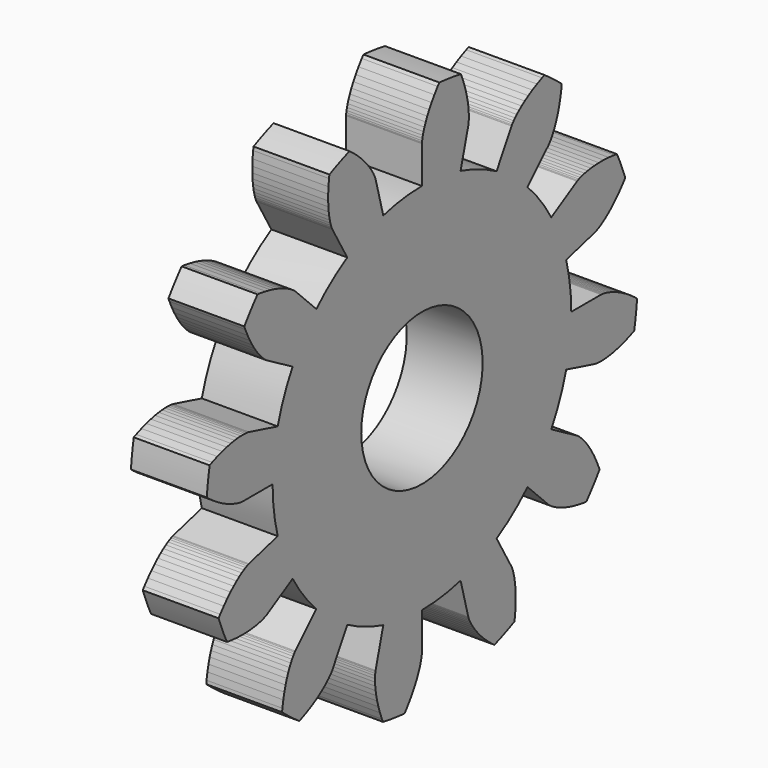
from build123d import *

# Parameters (mm, degrees)
F2_DEPTH = 5
F3_R     = 5
F4_DEPTH = 5.001


# Not quite as in the source:
# - a feature names something its author has since deleted; it is built from what else it names


with BuildPart() as f2:
    # F1 (on Right) → F2 (new body)
    with BuildSketch(Plane.YZ):
        with BuildLine():
            ThreePointArc((11.8820660929, -3.183790014), (12.1959813576, -1.6056314063), (12.30122, 0))
            ThreePointArc((12.30122, 0), (12.1959813576, 1.6056314063), (11.8820660929, 3.183790014))
            ThreePointArc((11.8820660929, 3.183790014), (11.3648453829, 4.7074730919), (10.6531690175, 6.15061))
            ThreePointArc((10.6531690175, 6.15061), (9.7592139767, 7.4885082658), (8.6982760789, 8.6982760789))
            ThreePointArc((8.6982760789, 8.6982760789), (7.4885082658, 9.7592139767), (6.15061, 10.6531690175))
            ThreePointArc((6.15061, 10.6531690175), (4.7074730919, 11.3648453829), (3.183790014, 11.8820660929))
            ThreePointArc((3.183790014, 11.8820660929), (1.6056314063, 12.1959813576), (0, 12.30122))
            ThreePointArc((0, 12.30122), (-1.6056314063, 12.1959813576), (-3.183790014, 11.8820660929))
            ThreePointArc((-3.183790014, 11.8820660929), (-4.7074730919, 11.3648453829), (-6.15061, 10.6531690175))
            ThreePointArc((-6.15061, 10.6531690175), (-7.4885082658, 9.7592139767), (-8.6982760789, 8.6982760789))
            ThreePointArc((-8.6982760789, 8.6982760789), (-9.7592139767, 7.4885082658), (-10.6531690175, 6.15061))
            ThreePointArc((-10.6531690175, 6.15061), (-11.3648453829, 4.7074730919), (-11.8820660929, 3.183790014))
            ThreePointArc((-11.8820660929, 3.183790014), (-12.1959813576, 1.6056314063), (-12.30122, 0))
            ThreePointArc((-12.30122, 0), (-12.1959813576, -1.6056314063), (-11.8820660929, -3.183790014))
            ThreePointArc((-11.8820660929, -3.183790014), (-11.3648453829, -4.7074730919), (-10.6531690175, -6.15061))
            ThreePointArc((-10.6531690175, -6.15061), (-9.7592139767, -7.4885082658), (-8.6982760789, -8.6982760789))
            ThreePointArc((-8.6982760789, -8.6982760789), (-7.4885082658, -9.7592139767), (-6.15061, -10.6531690175))
            ThreePointArc((-6.15061, -10.6531690175), (-4.7074730919, -11.3648453829), (-3.183790014, -11.8820660929))
            ThreePointArc((-3.183790014, -11.8820660929), (-1.6056314063, -12.1959813576), (0, -12.30122))
            ThreePointArc((0, -12.30122), (1.6056314063, -12.1959813576), (3.183790014, -11.8820660929))
            ThreePointArc((3.183790014, -11.8820660929), (4.7074730919, -11.3648453829), (6.15061, -10.6531690175))
            ThreePointArc((6.15061, -10.6531690175), (7.4885082658, -9.7592139767), (8.6982760789, -8.6982760789))
            ThreePointArc((8.6982760789, -8.6982760789), (9.7592139767, -7.4885082658), (10.6531690175, -6.15061))
            ThreePointArc((10.6531690175, -6.15061), (11.3648453829, -4.7074730919), (11.8820660929, -3.183790014))
        make_face()
        with BuildLine():
            Line((-12.777832476, -7.3772850197), (-10.6531690175, -6.15061))
            ThreePointArc((-10.6531690175, -6.15061), (-11.3648453829, -4.7074730919), (-11.8820660929, -3.183790014))
            Line((-11.8820660929, -3.183790014), (-14.2518202568, -3.8187637285))
            Line((-14.2518202568, -3.8187637285), (-14.2694648269, -3.824127867))
            Line((-14.2694648269, -3.824127867), (-14.3216296662, -3.8425556758))
            Line((-14.3216296662, -3.8425556758), (-14.4069660463, -3.8774806861))
            Line((-14.4069660463, -3.8774806861), (-14.5238699427, -3.9322299545))
            Line((-14.5238699427, -3.9322299545), (-14.6704895203, -4.0100072128))
            Line((-14.6704895203, -4.0100072128), (-14.84473366, -4.1138765105))
            Line((-14.84473366, -4.1138765105), (-15.0442814965, -4.2467464121))
            Line((-15.0442814965, -4.2467464121), (-15.2665929313, -4.4113548082))
            Line((-15.2665929313, -4.4113548082), (-15.5089200841, -4.6102543989))
            Line((-15.5089200841, -4.6102543989), (-15.7683196404, -4.8457989047))
            Line((-15.7683196404, -4.8457989047), (-16.0416660512, -5.1201300574))
            Line((-16.0416660512, -5.1201300574), (-16.3256655366, -5.4351654226))
            Line((-16.3256655366, -5.4351654226), (-16.616870844, -5.7925870994))
            Line((-16.616870844, -5.7925870994), (-16.7475876092, -5.9704865189))
            ThreePointArc((-16.7475876092, -5.9704865189), (-16.4265780881, -6.8041114275), (-16.0641042715, -7.6205612624))
            Line((-16.0641042715, -7.6205612624), (-15.8458796744, -7.6539244373))
            Line((-15.8458796744, -7.6539244373), (-15.3872311355, -7.7007464811))
            Line((-15.3872311355, -7.7007464811), (-14.9636495305, -7.7226921621))
            Line((-14.9636495305, -7.7226921621), (-14.5763830115, -7.7233884799))
            Line((-14.5763830115, -7.7233884799), (-14.2264047088, -7.7065204119))
            Line((-14.2264047088, -7.7065204119), (-13.9144102864, -7.6758124883))
            Line((-13.9144102864, -7.6758124883), (-13.6408166502, -7.6350102783))
            Line((-13.6408166502, -7.6350102783), (-13.4057618135, -7.5878618584))
            Line((-13.4057618135, -7.5878618584), (-13.2091059159, -7.5380993303))
            Line((-13.2091059159, -7.5380993303), (-13.0504333916, -7.4894204595))
            Line((-13.0504333916, -7.4894204595), (-12.9290562747, -7.4454705006))
            Line((-12.9290562747, -7.4454705006), (-12.84401863, -7.4098242792))
            Line((-12.84401863, -7.4098242792), (-12.7941020899, -7.3859685961))
            Line((-12.7941020899, -7.3859685961), (-12.777832476, -7.3772850197))
        make_face()
        with BuildLine():
            Line((-7.3772850197, -12.777832476), (-6.15061, -10.6531690175))
            ThreePointArc((-6.15061, -10.6531690175), (-7.4885082658, -9.7592139767), (-8.6982760789, -8.6982760789))
            Line((-8.6982760789, -8.6982760789), (-10.4330565283, -10.4330565283))
            Line((-10.4330565283, -10.4330565283), (-10.445655105, -10.4465242936))
            Line((-10.445655105, -10.4465242936), (-10.4816172766, -10.4885656638))
            Line((-10.4816172766, -10.4885656638), (-10.5380582445, -10.5614798))
            Line((-10.5380582445, -10.5614798), (-10.6119253544, -10.6673460055))
            Line((-10.6119253544, -10.6673460055), (-10.7000130041, -10.8080128758))
            Line((-10.7000130041, -10.8080128758), (-10.7989782067, -10.9850883961))
            Line((-10.7989782067, -10.9850883961), (-10.9053567516, -11.1999310245))
            Line((-10.9053567516, -11.1999310245), (-11.0155799037, -11.4536417946))
            Line((-11.0155799037, -11.4536417946), (-11.1259915786, -11.7470574694))
            Line((-11.1259915786, -11.7470574694), (-11.2328659313, -12.0807447733))
            Line((-11.2328659313, -12.0807447733), (-11.3324252906, -12.454995726))
            Line((-11.3324252906, -12.454995726), (-11.4208583771, -12.869824098))
            Line((-11.4208583771, -12.869824098), (-11.4943387326, -13.3249630037))
            Line((-11.4943387326, -13.3249630037), (-11.5185930622, -13.5443868029))
            ThreePointArc((-11.5185930622, -13.5443868029), (-10.8237782078, -14.1058223904), (-10.1016417569, -14.6316517801))
            Line((-10.1016417569, -14.6316517801), (-9.8959721247, -14.5514328385))
            Line((-9.8959721247, -14.5514328385), (-9.4753598166, -14.3626576485))
            Line((-9.4753598166, -14.3626576485), (-9.0975545457, -14.1698723633))
            Line((-9.0975545457, -14.1698723633), (-8.7618237433, -13.9768421326))
            Line((-8.7618237433, -13.9768421326), (-8.4671676764, -13.7872448059))
            Line((-8.4671676764, -13.7872448059), (-8.2123265426, -13.6046537527))
            Line((-8.2123265426, -13.6046537527), (-7.9957886083, -13.4325211843))
            Line((-7.9957886083, -13.4325211843), (-7.8157993584, -13.2741620365))
            Line((-7.8157993584, -13.2741620365), (-7.6703716193, -13.1327384743))
            Line((-7.6703716193, -13.1327384743), (-7.5572966178, -13.0112450734))
            Line((-7.5572966178, -13.0112450734), (-7.4741559306, -12.912494734))
            Line((-7.4741559306, -12.912494734), (-7.4183342807, -12.8391053784))
            Line((-7.4183342807, -12.8391053784), (-7.3870331304, -12.7934874807))
            Line((-7.3870331304, -12.7934874807), (-7.3772850197, -12.777832476))
        make_face()
        with BuildLine():
            Line((0, -14.7545700394), (0, -12.30122))
            ThreePointArc((0, -12.30122), (-1.6056314063, -12.1959813576), (-3.183790014, -11.8820660929))
            Line((-3.183790014, -11.8820660929), (-3.8187637285, -14.2518202568))
            Line((-3.8187637285, -14.2518202568), (-3.8229405333, -14.269782972))
            Line((-3.8229405333, -14.269782972), (-3.8330640024, -14.3241729524))
            Line((-3.8330640024, -14.3241729524), (-3.8454862463, -14.4155389306))
            Line((-3.8454862463, -14.4155389306), (-3.8565239372, -14.5441553089))
            Line((-3.8565239372, -14.5441553089), (-3.8624766445, -14.7100202169))
            Line((-3.8624766445, -14.7100202169), (-3.8596452639, -14.9128547172))
            Line((-3.8596452639, -14.9128547172), (-3.844350472, -15.1521031637))
            Line((-3.844350472, -15.1521031637), (-3.8129511367, -15.4269347118))
            Line((-3.8129511367, -15.4269347118), (-3.7618626147, -15.7362459776))
            Line((-3.7618626147, -15.7362459776), (-3.6875748671, -16.078664836))
            Line((-3.6875748671, -16.078664836), (-3.5866703252, -16.4525553481))
            Line((-3.5866703252, -16.4525553481), (-3.4558414386, -16.8560237997))
            Line((-3.4558414386, -16.8560237997), (-3.2919078403, -17.286925832))
            Line((-3.2919078403, -17.286925832), (-3.2032008062, -17.4890795811))
            ThreePointArc((-3.2032008062, -17.4890795811), (-2.3207556977, -17.6278896352), (-1.4324524914, -17.7222030194))
            Line((-1.4324524914, -17.7222030194), (-1.2944468359, -17.549896562))
            Line((-1.2944468359, -17.549896562), (-1.024573487, -17.1761062978))
            Line((-1.024573487, -17.1761062978), (-0.7937771672, -16.8202467078))
            Line((-0.7937771672, -16.8202467078), (-0.5995408789, -16.4852122232))
            Line((-0.5995408789, -16.4852122232), (-0.439159903, -16.1736880883))
            Line((-0.439159903, -16.1736880883), (-0.3097565337, -15.8881390309))
            Line((-0.3097565337, -15.8881390309), (-0.208295466, -15.6307988866))
            Line((-0.208295466, -15.6307988866), (-0.131599777, -15.4036612167))
            Line((-0.131599777, -15.4036612167), (-0.0763674416, -15.2084709496))
            Line((-0.0763674416, -15.2084709496), (-0.0391883182, -15.0467170773))
            Line((-0.0391883182, -15.0467170773), (-0.0165615407, -14.9196264312))
            Line((-0.0165615407, -14.9196264312), (-0.0049132517, -14.8281585599))
            Line((-0.0049132517, -14.8281585599), (-0.0006146092, -14.7730017265))
            Line((-0.0006146092, -14.7730017265), (0, -14.7545700394))
        make_face()
        with BuildLine():
            Line((7.3772850197, -12.777832476), (6.15061, -10.6531690175))
            ThreePointArc((6.15061, -10.6531690175), (4.7074730919, -11.3648453829), (3.183790014, -11.8820660929))
            Line((3.183790014, -11.8820660929), (3.8187637285, -14.2518202568))
            Line((3.8187637285, -14.2518202568), (3.824127867, -14.2694648269))
            Line((3.824127867, -14.2694648269), (3.8425556758, -14.3216296662))
            Line((3.8425556758, -14.3216296662), (3.8774806861, -14.4069660463))
            Line((3.8774806861, -14.4069660463), (3.9322299545, -14.5238699427))
            Line((3.9322299545, -14.5238699427), (4.0100072128, -14.6704895203))
            Line((4.0100072128, -14.6704895203), (4.1138765105, -14.84473366))
            Line((4.1138765105, -14.84473366), (4.2467464121, -15.0442814965))
            Line((4.2467464121, -15.0442814965), (4.4113548082, -15.2665929313))
            Line((4.4113548082, -15.2665929313), (4.6102543989, -15.5089200841))
            Line((4.6102543989, -15.5089200841), (4.8457989047, -15.7683196404))
            Line((4.8457989047, -15.7683196404), (5.1201300574, -16.0416660512))
            Line((5.1201300574, -16.0416660512), (5.4351654226, -16.3256655366))
            Line((5.4351654226, -16.3256655366), (5.7925870994, -16.616870844))
            Line((5.7925870994, -16.616870844), (5.9704865189, -16.7475876092))
            ThreePointArc((5.9704865189, -16.7475876092), (6.8041114275, -16.4265780881), (7.6205612624, -16.0641042715))
            Line((7.6205612624, -16.0641042715), (7.6539244373, -15.8458796744))
            Line((7.6539244373, -15.8458796744), (7.7007464811, -15.3872311355))
            Line((7.7007464811, -15.3872311355), (7.7226921621, -14.9636495305))
            Line((7.7226921621, -14.9636495305), (7.7233884799, -14.5763830115))
            Line((7.7233884799, -14.5763830115), (7.7065204119, -14.2264047088))
            Line((7.7065204119, -14.2264047088), (7.6758124883, -13.9144102864))
            Line((7.6758124883, -13.9144102864), (7.6350102783, -13.6408166502))
            Line((7.6350102783, -13.6408166502), (7.5878618584, -13.4057618135))
            Line((7.5878618584, -13.4057618135), (7.5380993303, -13.2091059159))
            Line((7.5380993303, -13.2091059159), (7.4894204595, -13.0504333916))
            Line((7.4894204595, -13.0504333916), (7.4454705006, -12.9290562747))
            Line((7.4454705006, -12.9290562747), (7.4098242792, -12.84401863))
            Line((7.4098242792, -12.84401863), (7.3859685961, -12.7941020899))
            Line((7.3859685961, -12.7941020899), (7.3772850197, -12.777832476))
        make_face()
        with BuildLine():
            Line((12.777832476, -7.3772850197), (10.6531690175, -6.15061))
            ThreePointArc((10.6531690175, -6.15061), (9.7592139767, -7.4885082658), (8.6982760789, -8.6982760789))
            Line((8.6982760789, -8.6982760789), (10.4330565283, -10.4330565283))
            Line((10.4330565283, -10.4330565283), (10.4465242936, -10.445655105))
            Line((10.4465242936, -10.445655105), (10.4885656638, -10.4816172766))
            Line((10.4885656638, -10.4816172766), (10.5614798, -10.5380582445))
            Line((10.5614798, -10.5380582445), (10.6673460055, -10.6119253544))
            Line((10.6673460055, -10.6119253544), (10.8080128758, -10.7000130041))
            Line((10.8080128758, -10.7000130041), (10.9850883961, -10.7989782067))
            Line((10.9850883961, -10.7989782067), (11.1999310245, -10.9053567516))
            Line((11.1999310245, -10.9053567516), (11.4536417946, -11.0155799037))
            Line((11.4536417946, -11.0155799037), (11.7470574694, -11.1259915786))
            Line((11.7470574694, -11.1259915786), (12.0807447733, -11.2328659313))
            Line((12.0807447733, -11.2328659313), (12.454995726, -11.3324252906))
            Line((12.454995726, -11.3324252906), (12.869824098, -11.4208583771))
            Line((12.869824098, -11.4208583771), (13.3249630037, -11.4943387326))
            Line((13.3249630037, -11.4943387326), (13.5443868029, -11.5185930622))
            ThreePointArc((13.5443868029, -11.5185930622), (14.1058223904, -10.8237782078), (14.6316517801, -10.1016417569))
            Line((14.6316517801, -10.1016417569), (14.5514328385, -9.8959721247))
            Line((14.5514328385, -9.8959721247), (14.3626576485, -9.4753598166))
            Line((14.3626576485, -9.4753598166), (14.1698723633, -9.0975545457))
            Line((14.1698723633, -9.0975545457), (13.9768421326, -8.7618237433))
            Line((13.9768421326, -8.7618237433), (13.7872448059, -8.4671676764))
            Line((13.7872448059, -8.4671676764), (13.6046537527, -8.2123265426))
            Line((13.6046537527, -8.2123265426), (13.4325211843, -7.9957886083))
            Line((13.4325211843, -7.9957886083), (13.2741620365, -7.8157993584))
            Line((13.2741620365, -7.8157993584), (13.1327384743, -7.6703716193))
            Line((13.1327384743, -7.6703716193), (13.0112450734, -7.5572966178))
            Line((13.0112450734, -7.5572966178), (12.912494734, -7.4741559306))
            Line((12.912494734, -7.4741559306), (12.8391053784, -7.4183342807))
            Line((12.8391053784, -7.4183342807), (12.7934874807, -7.3870331304))
            Line((12.7934874807, -7.3870331304), (12.777832476, -7.3772850197))
        make_face()
        with BuildLine():
            Line((14.7545700394, 0), (12.30122, 0))
            ThreePointArc((12.30122, 0), (12.1959813576, -1.6056314063), (11.8820660929, -3.183790014))
            Line((11.8820660929, -3.183790014), (14.2518202568, -3.8187637285))
            Line((14.2518202568, -3.8187637285), (14.269782972, -3.8229405333))
            Line((14.269782972, -3.8229405333), (14.3241729524, -3.8330640024))
            Line((14.3241729524, -3.8330640024), (14.4155389306, -3.8454862463))
            Line((14.4155389306, -3.8454862463), (14.5441553089, -3.8565239372))
            Line((14.5441553089, -3.8565239372), (14.7100202169, -3.8624766445))
            Line((14.7100202169, -3.8624766445), (14.9128547172, -3.8596452639))
            Line((14.9128547172, -3.8596452639), (15.1521031637, -3.844350472))
            Line((15.1521031637, -3.844350472), (15.4269347118, -3.8129511367))
            Line((15.4269347118, -3.8129511367), (15.7362459776, -3.7618626147))
            Line((15.7362459776, -3.7618626147), (16.078664836, -3.6875748671))
            Line((16.078664836, -3.6875748671), (16.4525553481, -3.5866703252))
            Line((16.4525553481, -3.5866703252), (16.8560237997, -3.4558414386))
            Line((16.8560237997, -3.4558414386), (17.286925832, -3.2919078403))
            Line((17.286925832, -3.2919078403), (17.4890795811, -3.2032008062))
            ThreePointArc((17.4890795811, -3.2032008062), (17.6278896352, -2.3207556977), (17.7222030194, -1.4324524914))
            Line((17.7222030194, -1.4324524914), (17.549896562, -1.2944468359))
            Line((17.549896562, -1.2944468359), (17.1761062978, -1.024573487))
            Line((17.1761062978, -1.024573487), (16.8202467078, -0.7937771672))
            Line((16.8202467078, -0.7937771672), (16.4852122232, -0.5995408789))
            Line((16.4852122232, -0.5995408789), (16.1736880883, -0.439159903))
            Line((16.1736880883, -0.439159903), (15.8881390309, -0.3097565337))
            Line((15.8881390309, -0.3097565337), (15.6307988866, -0.208295466))
            Line((15.6307988866, -0.208295466), (15.4036612167, -0.131599777))
            Line((15.4036612167, -0.131599777), (15.2084709496, -0.0763674416))
            Line((15.2084709496, -0.0763674416), (15.0467170773, -0.0391883182))
            Line((15.0467170773, -0.0391883182), (14.9196264312, -0.0165615407))
            Line((14.9196264312, -0.0165615407), (14.8281585599, -0.0049132517))
            Line((14.8281585599, -0.0049132517), (14.7730017265, -0.0006146092))
            Line((14.7730017265, -0.0006146092), (14.7545700394, 0))
        make_face()
        with BuildLine():
            ThreePointArc((10.6531690175, 6.15061), (11.3648453829, 4.7074730919), (11.8820660929, 3.183790014))
            Line((11.8820660929, 3.183790014), (14.2518202568, 3.8187637285))
            Line((14.2518202568, 3.8187637285), (14.2694648269, 3.824127867))
            Line((14.2694648269, 3.824127867), (14.3216296662, 3.8425556758))
            Line((14.3216296662, 3.8425556758), (14.4069660463, 3.8774806861))
            Line((14.4069660463, 3.8774806861), (14.5238699427, 3.9322299545))
            Line((14.5238699427, 3.9322299545), (14.6704895203, 4.0100072128))
            Line((14.6704895203, 4.0100072128), (14.84473366, 4.1138765105))
            Line((14.84473366, 4.1138765105), (15.0442814965, 4.2467464121))
            Line((15.0442814965, 4.2467464121), (15.2665929313, 4.4113548082))
            Line((15.2665929313, 4.4113548082), (15.5089200841, 4.6102543989))
            Line((15.5089200841, 4.6102543989), (15.7683196404, 4.8457989047))
            Line((15.7683196404, 4.8457989047), (16.0416660512, 5.1201300574))
            Line((16.0416660512, 5.1201300574), (16.3256655366, 5.4351654226))
            Line((16.3256655366, 5.4351654226), (16.616870844, 5.7925870994))
            Line((16.616870844, 5.7925870994), (16.7475876092, 5.9704865189))
            ThreePointArc((16.7475876092, 5.9704865189), (16.4265780881, 6.8041114275), (16.0641042715, 7.6205612624))
            Line((16.0641042715, 7.6205612624), (15.8458796744, 7.6539244373))
            Line((15.8458796744, 7.6539244373), (15.3872311355, 7.7007464811))
            Line((15.3872311355, 7.7007464811), (14.9636495305, 7.7226921621))
            Line((14.9636495305, 7.7226921621), (14.5763830115, 7.7233884799))
            Line((14.5763830115, 7.7233884799), (14.2264047088, 7.7065204119))
            Line((14.2264047088, 7.7065204119), (13.9144102864, 7.6758124883))
            Line((13.9144102864, 7.6758124883), (13.6408166502, 7.6350102783))
            Line((13.6408166502, 7.6350102783), (13.4057618135, 7.5878618584))
            Line((13.4057618135, 7.5878618584), (13.2091059159, 7.5380993303))
            Line((13.2091059159, 7.5380993303), (13.0504333916, 7.4894204595))
            Line((13.0504333916, 7.4894204595), (12.9290562747, 7.4454705006))
            Line((12.9290562747, 7.4454705006), (12.84401863, 7.4098242792))
            Line((12.84401863, 7.4098242792), (12.7941020899, 7.3859685961))
            Line((12.7941020899, 7.3859685961), (12.777832476, 7.3772850197))
            Line((12.777832476, 7.3772850197), (10.6531690175, 6.15061))
        make_face()
        with BuildLine():
            ThreePointArc((6.15061, 10.6531690175), (7.4885082658, 9.7592139767), (8.6982760789, 8.6982760789))
            Line((8.6982760789, 8.6982760789), (10.4330565283, 10.4330565283))
            Line((10.4330565283, 10.4330565283), (10.445655105, 10.4465242936))
            Line((10.445655105, 10.4465242936), (10.4816172766, 10.4885656638))
            Line((10.4816172766, 10.4885656638), (10.5380582445, 10.5614798))
            Line((10.5380582445, 10.5614798), (10.6119253544, 10.6673460055))
            Line((10.6119253544, 10.6673460055), (10.7000130041, 10.8080128758))
            Line((10.7000130041, 10.8080128758), (10.7989782067, 10.9850883961))
            Line((10.7989782067, 10.9850883961), (10.9053567516, 11.1999310245))
            Line((10.9053567516, 11.1999310245), (11.0155799037, 11.4536417946))
            Line((11.0155799037, 11.4536417946), (11.1259915786, 11.7470574694))
            Line((11.1259915786, 11.7470574694), (11.2328659313, 12.0807447733))
            Line((11.2328659313, 12.0807447733), (11.3324252906, 12.454995726))
            Line((11.3324252906, 12.454995726), (11.4208583771, 12.869824098))
            Line((11.4208583771, 12.869824098), (11.4943387326, 13.3249630037))
            Line((11.4943387326, 13.3249630037), (11.5185930622, 13.5443868029))
            ThreePointArc((11.5185930622, 13.5443868029), (10.8237782078, 14.1058223904), (10.1016417569, 14.6316517801))
            Line((10.1016417569, 14.6316517801), (9.8959721247, 14.5514328385))
            Line((9.8959721247, 14.5514328385), (9.4753598166, 14.3626576485))
            Line((9.4753598166, 14.3626576485), (9.0975545457, 14.1698723633))
            Line((9.0975545457, 14.1698723633), (8.7618237433, 13.9768421326))
            Line((8.7618237433, 13.9768421326), (8.4671676764, 13.7872448059))
            Line((8.4671676764, 13.7872448059), (8.2123265426, 13.6046537527))
            Line((8.2123265426, 13.6046537527), (7.9957886083, 13.4325211843))
            Line((7.9957886083, 13.4325211843), (7.8157993584, 13.2741620365))
            Line((7.8157993584, 13.2741620365), (7.6703716193, 13.1327384743))
            Line((7.6703716193, 13.1327384743), (7.5572966178, 13.0112450734))
            Line((7.5572966178, 13.0112450734), (7.4741559306, 12.912494734))
            Line((7.4741559306, 12.912494734), (7.4183342807, 12.8391053784))
            Line((7.4183342807, 12.8391053784), (7.3870331304, 12.7934874807))
            Line((7.3870331304, 12.7934874807), (7.3772850197, 12.777832476))
            Line((7.3772850197, 12.777832476), (6.15061, 10.6531690175))
        make_face()
        with BuildLine():
            ThreePointArc((0, 12.30122), (1.6056314063, 12.1959813576), (3.183790014, 11.8820660929))
            Line((3.183790014, 11.8820660929), (3.8187637285, 14.2518202568))
            Line((3.8187637285, 14.2518202568), (3.8229405333, 14.269782972))
            Line((3.8229405333, 14.269782972), (3.8330640024, 14.3241729524))
            Line((3.8330640024, 14.3241729524), (3.8454862463, 14.4155389306))
            Line((3.8454862463, 14.4155389306), (3.8565239372, 14.5441553089))
            Line((3.8565239372, 14.5441553089), (3.8624766445, 14.7100202169))
            Line((3.8624766445, 14.7100202169), (3.8596452639, 14.9128547172))
            Line((3.8596452639, 14.9128547172), (3.844350472, 15.1521031637))
            Line((3.844350472, 15.1521031637), (3.8129511367, 15.4269347118))
            Line((3.8129511367, 15.4269347118), (3.7618626147, 15.7362459776))
            Line((3.7618626147, 15.7362459776), (3.6875748671, 16.078664836))
            Line((3.6875748671, 16.078664836), (3.5866703252, 16.4525553481))
            Line((3.5866703252, 16.4525553481), (3.4558414386, 16.8560237997))
            Line((3.4558414386, 16.8560237997), (3.2919078403, 17.286925832))
            Line((3.2919078403, 17.286925832), (3.2032008062, 17.4890795811))
            ThreePointArc((3.2032008062, 17.4890795811), (2.3207556977, 17.6278896352), (1.4324524914, 17.7222030194))
            Line((1.4324524914, 17.7222030194), (1.2944468359, 17.549896562))
            Line((1.2944468359, 17.549896562), (1.024573487, 17.1761062978))
            Line((1.024573487, 17.1761062978), (0.7937771672, 16.8202467078))
            Line((0.7937771672, 16.8202467078), (0.5995408789, 16.4852122232))
            Line((0.5995408789, 16.4852122232), (0.439159903, 16.1736880883))
            Line((0.439159903, 16.1736880883), (0.3097565337, 15.8881390309))
            Line((0.3097565337, 15.8881390309), (0.208295466, 15.6307988866))
            Line((0.208295466, 15.6307988866), (0.131599777, 15.4036612167))
            Line((0.131599777, 15.4036612167), (0.0763674416, 15.2084709496))
            Line((0.0763674416, 15.2084709496), (0.0391883182, 15.0467170773))
            Line((0.0391883182, 15.0467170773), (0.0165615407, 14.9196264312))
            Line((0.0165615407, 14.9196264312), (0.0049132517, 14.8281585599))
            Line((0.0049132517, 14.8281585599), (0.0006146092, 14.7730017265))
            Line((0.0006146092, 14.7730017265), (0, 14.7545700394))
            Line((0, 14.7545700394), (0, 12.30122))
        make_face()
        with BuildLine():
            ThreePointArc((-6.15061, 10.6531690175), (-4.7074730919, 11.3648453829), (-3.183790014, 11.8820660929))
            Line((-3.183790014, 11.8820660929), (-3.8187637285, 14.2518202568))
            Line((-3.8187637285, 14.2518202568), (-3.824127867, 14.2694648269))
            Line((-3.824127867, 14.2694648269), (-3.8425556758, 14.3216296662))
            Line((-3.8425556758, 14.3216296662), (-3.8774806861, 14.4069660463))
            Line((-3.8774806861, 14.4069660463), (-3.9322299545, 14.5238699427))
            Line((-3.9322299545, 14.5238699427), (-4.0100072128, 14.6704895203))
            Line((-4.0100072128, 14.6704895203), (-4.1138765105, 14.84473366))
            Line((-4.1138765105, 14.84473366), (-4.2467464121, 15.0442814965))
            Line((-4.2467464121, 15.0442814965), (-4.4113548082, 15.2665929313))
            Line((-4.4113548082, 15.2665929313), (-4.6102543989, 15.5089200841))
            Line((-4.6102543989, 15.5089200841), (-4.8457989047, 15.7683196404))
            Line((-4.8457989047, 15.7683196404), (-5.1201300574, 16.0416660512))
            Line((-5.1201300574, 16.0416660512), (-5.4351654226, 16.3256655366))
            Line((-5.4351654226, 16.3256655366), (-5.7925870994, 16.616870844))
            Line((-5.7925870994, 16.616870844), (-5.9704865189, 16.7475876092))
            ThreePointArc((-5.9704865189, 16.7475876092), (-6.8041114275, 16.4265780881), (-7.6205612624, 16.0641042715))
            Line((-7.6205612624, 16.0641042715), (-7.6539244373, 15.8458796744))
            Line((-7.6539244373, 15.8458796744), (-7.7007464811, 15.3872311355))
            Line((-7.7007464811, 15.3872311355), (-7.7226921621, 14.9636495305))
            Line((-7.7226921621, 14.9636495305), (-7.7233884799, 14.5763830115))
            Line((-7.7233884799, 14.5763830115), (-7.7065204119, 14.2264047088))
            Line((-7.7065204119, 14.2264047088), (-7.6758124883, 13.9144102864))
            Line((-7.6758124883, 13.9144102864), (-7.6350102783, 13.6408166502))
            Line((-7.6350102783, 13.6408166502), (-7.5878618584, 13.4057618135))
            Line((-7.5878618584, 13.4057618135), (-7.5380993303, 13.2091059159))
            Line((-7.5380993303, 13.2091059159), (-7.4894204595, 13.0504333916))
            Line((-7.4894204595, 13.0504333916), (-7.4454705006, 12.9290562747))
            Line((-7.4454705006, 12.9290562747), (-7.4098242792, 12.84401863))
            Line((-7.4098242792, 12.84401863), (-7.3859685961, 12.7941020899))
            Line((-7.3859685961, 12.7941020899), (-7.3772850197, 12.777832476))
            Line((-7.3772850197, 12.777832476), (-6.15061, 10.6531690175))
        make_face()
        with BuildLine():
            ThreePointArc((-10.6531690175, 6.15061), (-9.7592139767, 7.4885082658), (-8.6982760789, 8.6982760789))
            Line((-8.6982760789, 8.6982760789), (-10.4330565283, 10.4330565283))
            Line((-10.4330565283, 10.4330565283), (-10.4465242936, 10.445655105))
            Line((-10.4465242936, 10.445655105), (-10.4885656638, 10.4816172766))
            Line((-10.4885656638, 10.4816172766), (-10.5614798, 10.5380582445))
            Line((-10.5614798, 10.5380582445), (-10.6673460055, 10.6119253544))
            Line((-10.6673460055, 10.6119253544), (-10.8080128758, 10.7000130041))
            Line((-10.8080128758, 10.7000130041), (-10.9850883961, 10.7989782067))
            Line((-10.9850883961, 10.7989782067), (-11.1999310245, 10.9053567516))
            Line((-11.1999310245, 10.9053567516), (-11.4536417946, 11.0155799037))
            Line((-11.4536417946, 11.0155799037), (-11.7470574694, 11.1259915786))
            Line((-11.7470574694, 11.1259915786), (-12.0807447733, 11.2328659313))
            Line((-12.0807447733, 11.2328659313), (-12.454995726, 11.3324252906))
            Line((-12.454995726, 11.3324252906), (-12.869824098, 11.4208583771))
            Line((-12.869824098, 11.4208583771), (-13.3249630037, 11.4943387326))
            Line((-13.3249630037, 11.4943387326), (-13.5443868029, 11.5185930622))
            ThreePointArc((-13.5443868029, 11.5185930622), (-14.1058223904, 10.8237782078), (-14.6316517801, 10.1016417569))
            Line((-14.6316517801, 10.1016417569), (-14.5514328385, 9.8959721247))
            Line((-14.5514328385, 9.8959721247), (-14.3626576485, 9.4753598166))
            Line((-14.3626576485, 9.4753598166), (-14.1698723633, 9.0975545457))
            Line((-14.1698723633, 9.0975545457), (-13.9768421326, 8.7618237433))
            Line((-13.9768421326, 8.7618237433), (-13.7872448059, 8.4671676764))
            Line((-13.7872448059, 8.4671676764), (-13.6046537527, 8.2123265426))
            Line((-13.6046537527, 8.2123265426), (-13.4325211843, 7.9957886083))
            Line((-13.4325211843, 7.9957886083), (-13.2741620365, 7.8157993584))
            Line((-13.2741620365, 7.8157993584), (-13.1327384743, 7.6703716193))
            Line((-13.1327384743, 7.6703716193), (-13.0112450734, 7.5572966178))
            Line((-13.0112450734, 7.5572966178), (-12.912494734, 7.4741559306))
            Line((-12.912494734, 7.4741559306), (-12.8391053784, 7.4183342807))
            Line((-12.8391053784, 7.4183342807), (-12.7934874807, 7.3870331304))
            Line((-12.7934874807, 7.3870331304), (-12.777832476, 7.3772850197))
            Line((-12.777832476, 7.3772850197), (-10.6531690175, 6.15061))
        make_face()
        with BuildLine():
            ThreePointArc((-12.30122, 0), (-12.1959813576, 1.6056314063), (-11.8820660929, 3.183790014))
            Line((-11.8820660929, 3.183790014), (-14.2518202568, 3.8187637285))
            Line((-14.2518202568, 3.8187637285), (-14.269782972, 3.8229405333))
            Line((-14.269782972, 3.8229405333), (-14.3241729524, 3.8330640024))
            Line((-14.3241729524, 3.8330640024), (-14.4155389306, 3.8454862463))
            Line((-14.4155389306, 3.8454862463), (-14.5441553089, 3.8565239372))
            Line((-14.5441553089, 3.8565239372), (-14.7100202169, 3.8624766445))
            Line((-14.7100202169, 3.8624766445), (-14.9128547172, 3.8596452639))
            Line((-14.9128547172, 3.8596452639), (-15.1521031637, 3.844350472))
            Line((-15.1521031637, 3.844350472), (-15.4269347118, 3.8129511367))
            Line((-15.4269347118, 3.8129511367), (-15.7362459776, 3.7618626147))
            Line((-15.7362459776, 3.7618626147), (-16.078664836, 3.6875748671))
            Line((-16.078664836, 3.6875748671), (-16.4525553481, 3.5866703252))
            Line((-16.4525553481, 3.5866703252), (-16.8560237997, 3.4558414386))
            Line((-16.8560237997, 3.4558414386), (-17.286925832, 3.2919078403))
            Line((-17.286925832, 3.2919078403), (-17.4890795811, 3.2032008062))
            ThreePointArc((-17.4890795811, 3.2032008062), (-17.6278896352, 2.3207556977), (-17.7222030194, 1.4324524914))
            Line((-17.7222030194, 1.4324524914), (-17.549896562, 1.2944468359))
            Line((-17.549896562, 1.2944468359), (-17.1761062978, 1.024573487))
            Line((-17.1761062978, 1.024573487), (-16.8202467078, 0.7937771672))
            Line((-16.8202467078, 0.7937771672), (-16.4852122232, 0.5995408789))
            Line((-16.4852122232, 0.5995408789), (-16.1736880883, 0.439159903))
            Line((-16.1736880883, 0.439159903), (-15.8881390309, 0.3097565337))
            Line((-15.8881390309, 0.3097565337), (-15.6307988866, 0.208295466))
            Line((-15.6307988866, 0.208295466), (-15.4036612167, 0.131599777))
            Line((-15.4036612167, 0.131599777), (-15.2084709496, 0.0763674416))
            Line((-15.2084709496, 0.0763674416), (-15.0467170773, 0.0391883182))
            Line((-15.0467170773, 0.0391883182), (-14.9196264312, 0.0165615407))
            Line((-14.9196264312, 0.0165615407), (-14.8281585599, 0.0049132517))
            Line((-14.8281585599, 0.0049132517), (-14.7730017265, 0.0006146092))
            Line((-14.7730017265, 0.0006146092), (-14.7545700394, 0))
            Line((-14.7545700394, 0), (-12.30122, 0))
        make_face()
    extrude(amount=F2_DEPTH)

    # F3 (on face) → F4 (cut, through all)
    with BuildSketch(Plane(origin=(0, 0, 0), x_dir=(0, -1, 0), z_dir=(-1, 0, 0))):
        Circle(F3_R)
    extrude(amount=-F4_DEPTH, mode=Mode.SUBTRACT)


solid = f2.part
